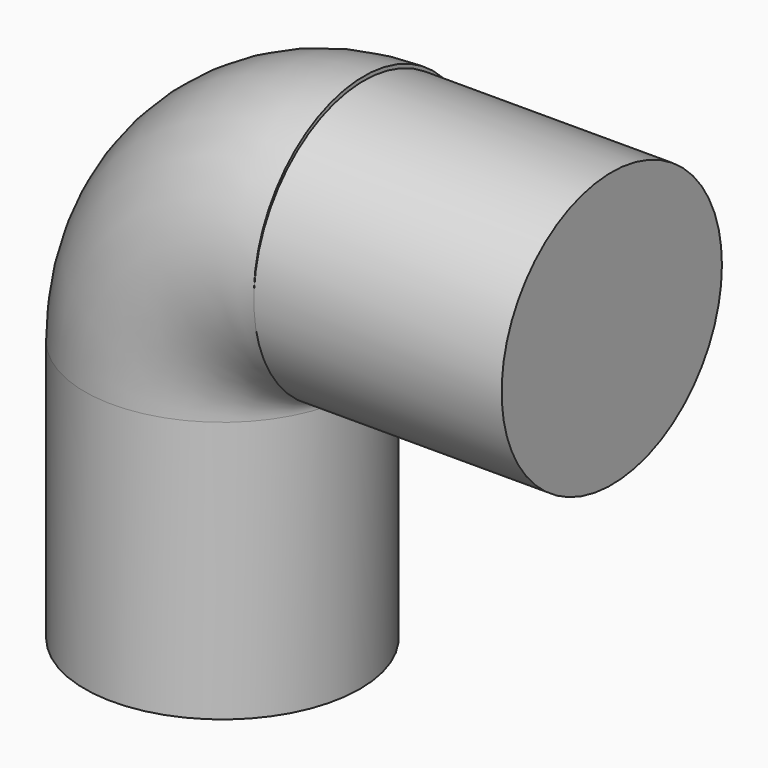
from build123d import *

# Parameters (mm, degrees)
F1_R      = 10
F2_DEPTH  = 18
F0_R      = 10
F3_DEPTH  = 19
F3_FACE_R = 10
F5_ANGLE  = 90


with BuildPart() as f2:
    # F1 (on Right) → F2 (new body)
    with BuildSketch(Plane.YZ):
        with Locations((10, 10)):
            Circle(F1_R)
    extrude(amount=-F2_DEPTH)


with BuildPart() as f3:
    # F0 (on Top) → F3 (new body)
    with BuildSketch(Plane.XY):
        with Locations((-28.2842712475, 10)):
            Circle(F0_R)
    extrude(amount=-F3_DEPTH)

    # F3_face (on face) → F5 (revolve)
    with BuildSketch(Plane(origin=(-28.2842712475, 10, 0), x_dir=(1, 0, 0), z_dir=(0, 0, 1))):
        Circle(F3_FACE_R)
    revolve(axis=Axis((-18, 7.3859319091, 0), (0, 1, 0)), revolution_arc=F5_ANGLE)


solid = Compound([f2.part, f3.part])
